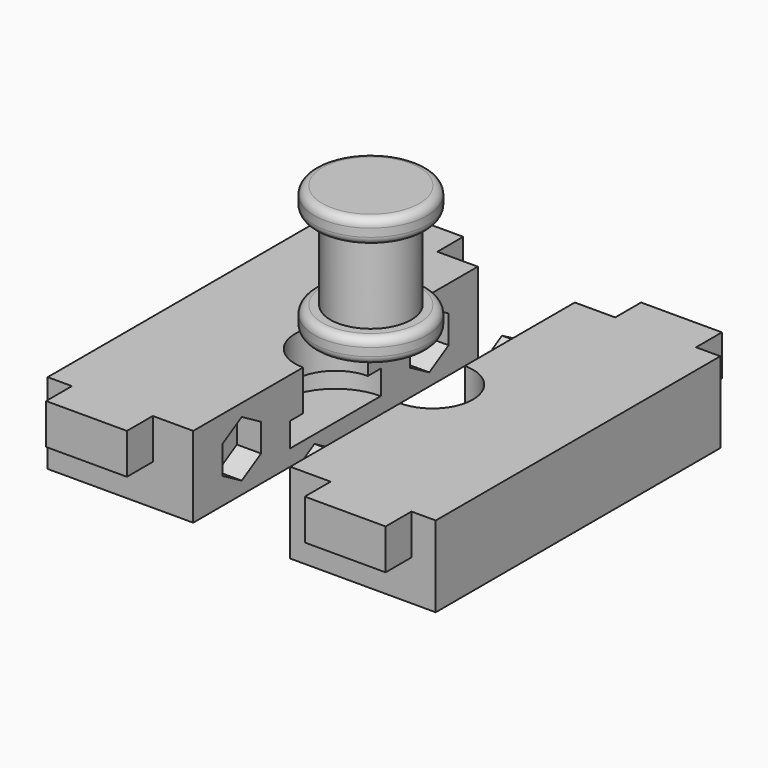
from build123d import *

# Parameters (mm, degrees)
F0_W      = 9
F0_H      = 22
F0_W_2    = 4
F0_H_2    = 5
F1_DEPTH  = 5
F2_DEPTH  = 2
F4_DEPTH  = 4
F5_DEPTH  = 2.5
F7_DEPTH  = 1.5
F8_W      = 5
F8_H      = 2.5
F9_DEPTH  = 2
F13_DEPTH = 3
F16_R     = 0.5


# Not quite as in the source:
# - a pattern or mirror of a feature is missing from the dataset's text; its kind, count and spacing are read off the source's solid


with BuildPart() as f1:
    # F0 (on Top) → F1 (new body)
    with BuildSketch(Plane.XY):
        with Locations((4.5, 10)):
            Rectangle(F0_W, F0_H)
        with Locations((5, 2.5)):
            Rectangle(F0_W_2, F0_H_2, mode=Mode.SUBTRACT)
        with Locations((5, 17.5)):
            Rectangle(F0_W_2, F0_H_2, mode=Mode.SUBTRACT)
        with Locations((5, 17.5)):
            Rectangle(F0_W_2, F0_H_2)
        with Locations((5, 2.5)):
            Rectangle(F0_W_2, F0_H_2)
    extrude(amount=F1_DEPTH)

    # F0 (on Top) → F2 (cut)
    with BuildSketch(Plane.XY):
        with Locations((5, 2.5)):
            Rectangle(F0_W_2, F0_H_2)
        with Locations((5, 17.5)):
            Rectangle(F0_W_2, F0_H_2)
    extrude(amount=F2_DEPTH, mode=Mode.SUBTRACT)

    # F3 (on face) → F4 (cut)
    with BuildSketch(Plane.XY.offset(5)):
        with BuildLine():
            Line((9, 12.5), (9, 13.5))
            ThreePointArc((9, 13.5), (5.5, 10), (9, 6.5))
            Line((9, 6.5), (9, 7.5))
            ThreePointArc((9, 7.5), (6.5, 10), (9, 12.5))
        make_face()
        with BuildLine():
            Line((9, 7.5), (9, 12.5))
            ThreePointArc((9, 12.5), (6.5, 10), (9, 7.5))
        make_face()
    extrude(amount=-F4_DEPTH, mode=Mode.SUBTRACT)

    # F3 (on face) → F5 (join)
    with BuildSketch(Plane.XY.offset(5)):
        with BuildLine():
            Line((9, 12.5), (9, 13.5))
            ThreePointArc((9, 13.5), (5.5, 10), (9, 6.5))
            Line((9, 6.5), (9, 7.5))
            ThreePointArc((9, 7.5), (6.5, 10), (9, 12.5))
        make_face()
    extrude(amount=-F5_DEPTH)

    # F6 (on face) → F7 (cut)
    with BuildSketch(Plane.YZ.offset(9)):
        Polygon((1.25, 3.3660254038), (1.25, 1.6339745962), (2.75, 0.7679491924), (4.25, 1.6339745962), (4.25, 3.3660254038), (2.75, 4.2320508076), align=None)
        Polygon((18.75, 1.6339745962), (18.75, 3.3660254038), (17.25, 4.2320508076), (15.75, 3.3660254038), (15.75, 1.6339745962), (17.25, 0.7679491924), align=None)
    extrude(amount=-F7_DEPTH, mode=Mode.SUBTRACT)

    # F8 (on face) → F9 (join)
    with BuildSketch(Plane(origin=(0, 21, 0), x_dir=(-1, 0, 0), z_dir=(0, 1, 0))):
        with Locations((-4, 3.75)):
            Rectangle(F8_W, F8_H)
    f9 = extrude(amount=F9_DEPTH)

    # F9_copies: F9 across plane
    add(f9.mirror(Plane(origin=(0, 10, 0), x_dir=(0, 0, -1), z_dir=(0, -1, 0))))


with BuildPart() as f12_1:
    # F12: instance of F1
    add(f1.part.mirror(Plane.YZ.offset(12)))

    # F13 (add): faces of the model
    f13_faces = [f12_1.faces().sort_by_distance(p)[0] for p in [
        (16.5, 2.75, 2.5),
        (16.5, 17.25, 2.5),
    ]]
    extrude(f13_faces, amount=F13_DEPTH)


with BuildPart() as f15:
    # F14 (on offset) → F15 (revolve)
    with BuildSketch(Plane.XZ.offset(-10)):
        Polygon((7.6874490976, 6.599618122), (11.1874490976, 6.599618122), (11.1874490976, 14.599618122), (7.6874490976, 14.599618122), (7.6874490976, 13.099618122), (8.6874490976, 13.099618122), (8.6874490976, 10.599618122), (8.6874490976, 8.099618122), (7.6874490976, 8.099618122), align=None)
    revolve(axis=Axis((11.1874490976, 10, 10.599618122), (0, 0, -1)))

    # F16
    f16_edges = [f15.edges().sort_by_distance(p)[0] for p in [
        (14.687449, 10, 14.599618),
        (14.687449, 10, 8.099618),
        (14.687449, 10, 13.099618),
        (7.687449, 10, 13.849618),
        (14.687449, 10, 6.599618),
        (7.687449, 10, 7.349618),
    ]]
    fillet(f16_edges, radius=F16_R)


solid = Compound([f1.part, f12_1.part, f15.part])
